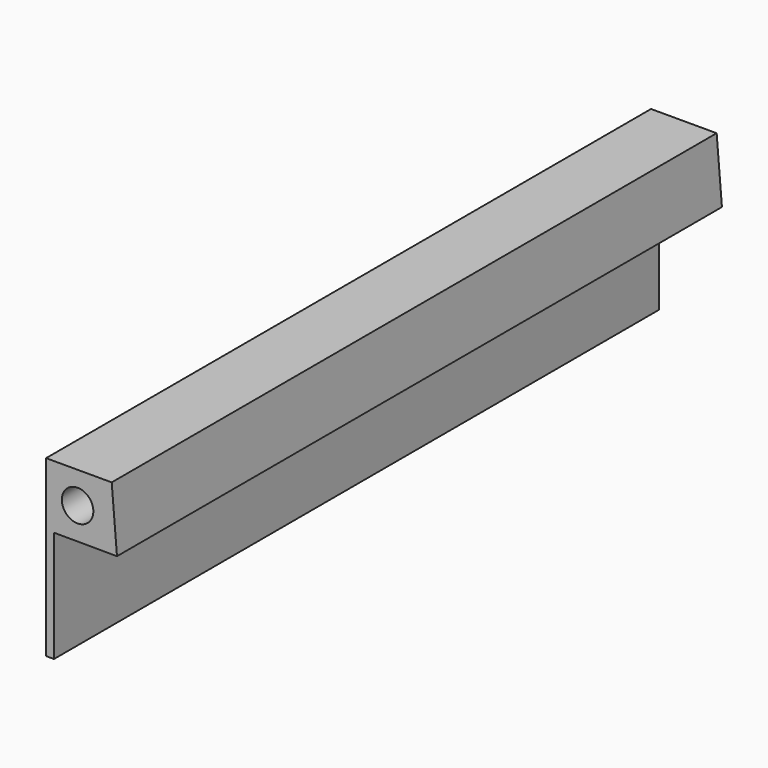
from build123d import *

# Parameters (mm, degrees)
F0_R     = 6.35
F1_DEPTH = 304.8


# Not quite as in the source:
# - a feature names something its author has since deleted; it is built from what else it names


with BuildPart() as f1:
    # F0 (on Front) → F1 (new body)
    with BuildSketch(Plane.XZ):
        Polygon((-9.525, -12.7128391741), (-12.7, -12.7), (-12.7, -57.5586806671), (-9.525, -57.5586806671), align=None)
        Polygon((15.8747663651, -12.8155516218), (13.7463785204, 12.7), (-12.7, 12.7), (-12.7, -12.7), (-9.525, -12.7), (-9.525, -12.7128391741), align=None)
        Circle(F0_R, mode=Mode.SUBTRACT)
        Polygon((-9.525, -12.7), (-12.7, -12.7), (-9.525, -12.7128391741), align=None)
    extrude(amount=F1_DEPTH)


solid = f1.part
